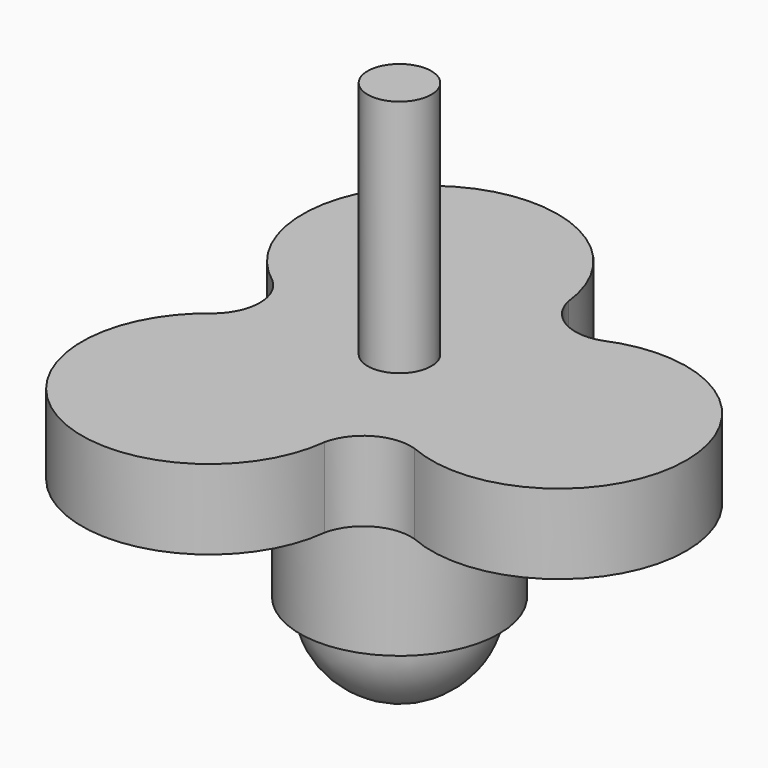
from build123d import *

# Parameters (mm, degrees)
F0_R     = 1.95
F1_DEPTH = 5
F2_R     = 6.25
F3_DEPTH = 3.2
F4_R     = 6.25
F4_R_2   = 5.25
F5_DEPTH = 5.2
F6_R     = 2
F7_DEPTH = 15


# Not quite as in the source:
# - ends of sketch curves that miss each other by under 0.0002 mm in the source are joined


with BuildPart() as f1:
    # F0 (on Top) → F1 (new body)
    with BuildSketch(Plane.XY):
        with BuildLine():
            ThreePointArc((2.9498031466, -9.5550333017), (4.3822075591, -7.5902061417), (6.8, -7.3321211119))
            ThreePointArc((6.8, -7.3321211119), (18, 0), (6.8, 7.3321211119))
            ThreePointArc((6.8, 7.3321211119), (4.3822075591, 7.5902061417), (2.9498031466, 9.5550333017))
            ThreePointArc((2.9498031466, 9.5550333017), (-9, 15.5884572681), (-9.7498031466, 2.2229121898))
            ThreePointArc((-9.7498031466, 2.2229121898), (-8.7644151183, 0), (-9.7498031466, -2.2229121898))
            ThreePointArc((-9.7498031466, -2.2229121898), (-9, -15.5884572681), (2.9498031466, -9.5550333017))
        make_face()
        Circle(F0_R, mode=Mode.SUBTRACT)
    extrude(amount=F1_DEPTH)

    # F6 (on face) → F7 (join)
    with BuildSketch(Plane.XY.offset(5)):
        Circle(F6_R)
    extrude(amount=F7_DEPTH)


with BuildPart() as f3:
    # F2 (on Top) → F3 (new body)
    with BuildSketch(Plane.XY):
        Circle(F2_R)
        Polygon((-1.5568529045, 4.0405703847), (2.7208101467, 3.3685593576), (4.2776630512, -0.6720110271), (1.5568529045, -4.0405703847), (-2.7208101467, -3.3685593576), (-4.2776630512, 0.6720110271), align=None, mode=Mode.SUBTRACT)
    extrude(amount=-F3_DEPTH)

    # F4 (on face) → F5 (join)
    with BuildSketch(Plane(origin=(0, 0, -3.2), x_dir=(1, 0, 0), z_dir=(0, 0, -1))):
        Circle(F4_R)
        Circle(F4_R_2, mode=Mode.SUBTRACT)
    extrude(amount=F5_DEPTH)


with BuildPart() as f9:
    # F8 (on face) → F9 (revolve)
    with BuildSketch(Plane(origin=(0, 0, -8.4), x_dir=(1, 0, 0), z_dir=(0, 0, -1))):
        with BuildLine():
            ThreePointArc((5.2500002044, 0), (0, 5.2500002044), (-5.2500002044, 0))
            Line((-5.2500002044, 0), (5.2500002044, 0))
        make_face()
    revolve(axis=Axis((0, 0, -8.4), (1, 0, 0)))


solid = Compound([f1.part, f3.part, f9.part])
